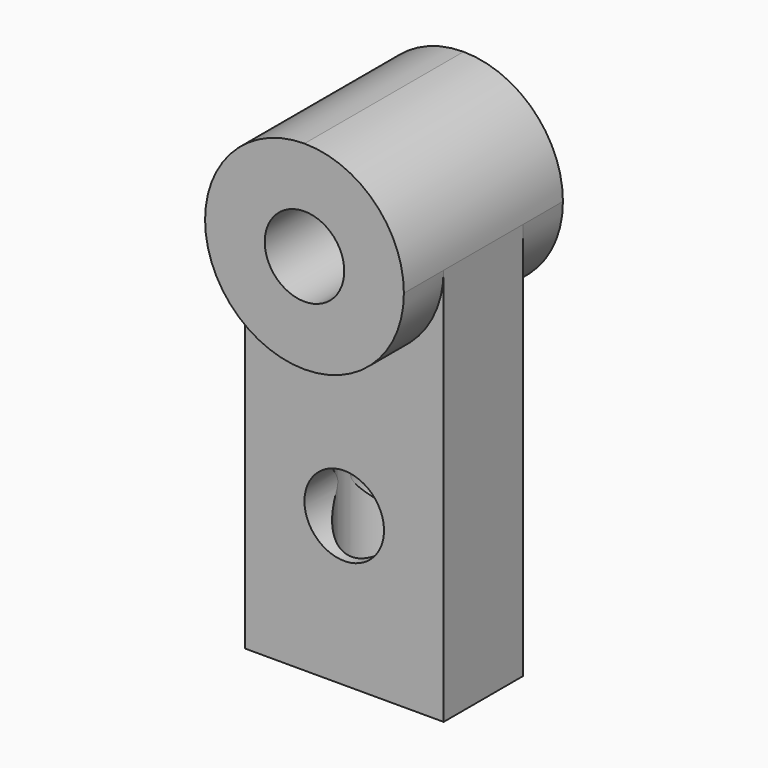
from build123d import *

# Parameters (mm, degrees)
F0_W          = 20
F0_H          = 50
F0_R          = 4
F1_DEPTH      = 10
F1_DEPTH_BACK = 10
F2_R          = 9.99999
F3_R          = 4.08
F4_DEPTH      = 20
F6_D          = 8
F7_R          = 4
F8_DEPTH      = 5


# Not quite as in the source:
# - a fillet or chamfer is up to 0.001 mm smaller than in the source, because OpenCascade refuses the exact size
# - ends of sketch curves that miss each other by under 0.0002 mm in the source are joined
# - a pattern or mirror of a feature is missing from the dataset's text; its kind, count and spacing are read off the source's solid


with BuildPart() as f1:
    # F0 (on Front) → F1 (new body, two sides)
    with BuildSketch(Plane.XZ) as f1_sk:
        with Locations((0, -10)):
            Rectangle(F0_W, F0_H)
        with Locations((0, 5)):
            Circle(F0_R, mode=Mode.SUBTRACT)
    extrude(amount=F1_DEPTH)
    extrude(f1_sk.sketch, amount=-F1_DEPTH_BACK)

    # F2 (radius 10 in the source; OpenCascade refuses exactly that, so slightly less here)
    f2_edges = [f1.edges().sort_by_distance(p)[0] for p in [
        (-10, 0, 15),
        (10, 0, 15),
    ]]
    fillet(f2_edges, radius=F2_R)

    # F3 (on face) → F4 (cut)
    with BuildSketch(Plane(origin=(0, 0, -35), x_dir=(1, 0, 0), z_dir=(0, 0, -1))):
        Circle(F3_R)
    extrude(amount=-F4_DEPTH, mode=Mode.SUBTRACT)

    # F6 (through all)
    with Locations(Plane.XZ.offset(10)):
        with Locations((0, -20)):
            Hole(F6_D / 2)

    # F7 (on face) → F8 (cut)
    with BuildSketch(Plane.XZ.offset(10)):
        with BuildLine():
            Line((10, -35), (10, 5))
            ThreePointArc((10, 5), (-2.5e-06, -5), (-10, 5.000005))
            Line((-10, 5.000005), (-10, -35))
            Line((-10, -35), (10, -35))
        make_face()
        with Locations((0, -20)):
            Circle(F7_R, mode=Mode.SUBTRACT)
    f8 = extrude(amount=-F8_DEPTH, mode=Mode.SUBTRACT)

    # F8_copies: F8 across plane
    add(f8.mirror(Plane.ZX), mode=Mode.SUBTRACT)


solid = f1.part
